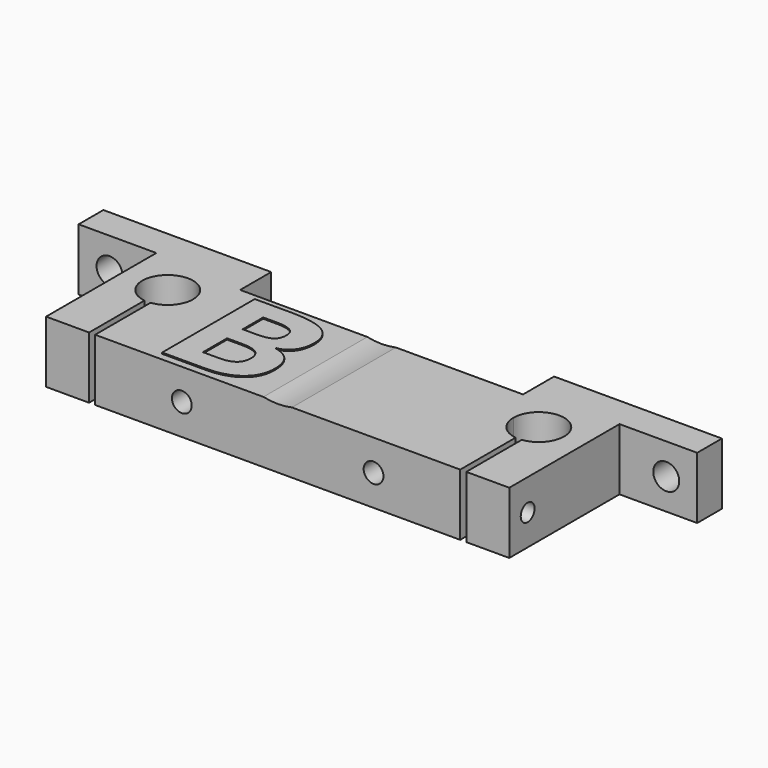
from build123d import *

# Parameters (mm, degrees)
F1_DEPTH      = 10
F2_R          = 1.6
F2_R_2        = 10.75
F3_DEPTH      = 27.2759499461
F4_R          = 2.1
F5_DEPTH      = 5.001
F7_DEPTH      = 10.001
F8_R          = 1.4
F9_DEPTH      = 18
F11_TEXT_SIZE = 26.2005653077
F12_DEPTH     = 0.2
F8_R_2        = 1.7
F13_DEPTH     = 6.9528983364


# Not quite as in the source:
# - Text() gives the source's letters only with a copy of the font that has no kerning and outlines rounded to 1/6400 em; it was checked with that copy


with BuildPart() as f1:
    # F0 (on Top) → F1 (new body)
    with BuildSketch(Plane.XY):
        Polygon((-37.4418646097, -13.8158900663), (0, -13.8158900663), (0, 7.1841099337), (-22.8655805642, 7.1841099337), (-22.8655805642, 13.4590598798), (-50, 13.4590598798), (-50, 8.4590598798), (-37.4418646097, 8.4590598798), align=None)
    extrude(amount=F1_DEPTH)

    # F2 (on face) → F3 (cut, through all)
    with BuildSketch(Plane.XZ.offset(13.8158900663)):
        with Locations((-15.5, 5)):
            Circle(F2_R)
        with Locations((0, 20.5)):
            Circle(F2_R_2)
    extrude(amount=-F3_DEPTH, mode=Mode.SUBTRACT)

    # F4 (on face) → F5 (cut, through all)
    with BuildSketch(Plane.XZ.offset(-8.4590598798)):
        with Locations((-45, 5)):
            Circle(F4_R)
    extrude(amount=-F5_DEPTH, mode=Mode.SUBTRACT)

    # F6 (on face) → F7 (cut, through all)
    with BuildSketch(Plane.XY.offset(10)):
        with BuildLine():
            ThreePointArc((-29.5100337267, -2.6115583842), (-26.9325204385, -1.2613388299), (-25.9, 1.4590598798))
            ThreePointArc((-25.9, 1.4590598798), (-32.7203987097, 4.5265394413), (-30.4899662733, -2.6115583842))
            Line((-30.4899662733, -2.6115583842), (-30.4899662733, -2.0438153297))
            Line((-30.4899662733, -2.0438153297), (-29.5100337267, -2.0438153297))
            Line((-29.5100337267, -2.0438153297), (-29.5100337267, -2.6115583842))
        make_face()
        with BuildLine():
            Line((-30.4899662733, -2.0438153297), (-30.4899662733, -2.6115583842))
            ThreePointArc((-30.4899662733, -2.6115583842), (-30, -2.6409401202), (-29.5100337267, -2.6115583842))
            Line((-29.5100337267, -2.6115583842), (-29.5100337267, -2.0438153297))
            Line((-29.5100337267, -2.0438153297), (-30.4899662733, -2.0438153297))
        make_face()
        with BuildLine():
            ThreePointArc((-29.5100337267, -2.6115583842), (-30, -2.6409401202), (-30.4899662733, -2.6115583842))
            Line((-30.4899662733, -2.6115583842), (-30.4899662733, -14.1640976071))
            Line((-30.4899662733, -14.1640976071), (-29.5100337267, -14.1640976071))
            Line((-29.5100337267, -14.1640976071), (-29.5100337267, -2.6115583842))
        make_face()
    extrude(amount=-F7_DEPTH, mode=Mode.SUBTRACT)

    # F8 (on face) → F9 (cut)
    with BuildSketch(Plane(origin=(-37.4418646097, 0, 0), x_dir=(0, -1, 0), z_dir=(-1, 0, 0))):
        with Locations((10.1014729589, 4.9766320735)):
            Circle(F8_R)
    extrude(amount=-F9_DEPTH, mode=Mode.SUBTRACT)

    # F10: F1 across plane


with BuildPart() as f1_1:
    add(f1.part)
    add(f1.part.mirror(Plane.YZ))

    # F11 (on face) → F12 (join)
    with BuildSketch(Plane.XY.offset(10)):
        with Locations((-21.9846321763, -12.614618754)):
            Text('B', F11_TEXT_SIZE, font='Open Sans', font_style=FontStyle.BOLD, text_align=(TextAlign.LEFT, TextAlign.BOTTOM))
    extrude(amount=F12_DEPTH)

    # F8 (on face) → F13 (cut, through all)
    with BuildSketch(Plane(origin=(-37.4418646097, 0, 0), x_dir=(0, -1, 0), z_dir=(-1, 0, 0))):
        with Locations((10.1014729589, 4.9766320735)):
            Circle(F8_R_2)
        with Locations((10.1014729589, 4.9766320735)):
            Circle(F8_R, mode=Mode.SUBTRACT)
        with Locations((10.1014729589, 4.9766320735)):
            Circle(F8_R)
    extrude(amount=-F13_DEPTH, mode=Mode.SUBTRACT)


solid = f1_1.part
